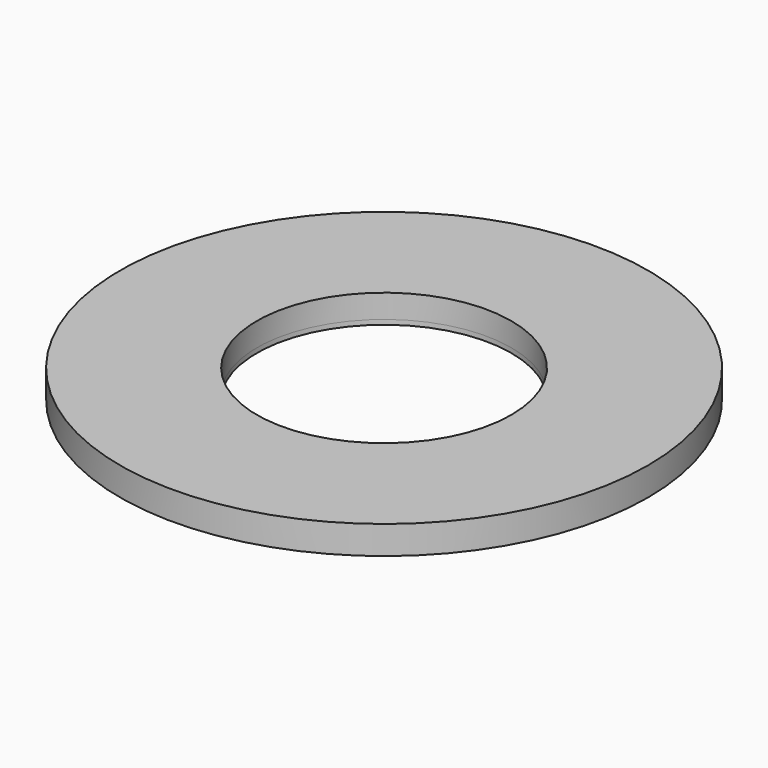
from build123d import *

# Parameters (mm, degrees)
F1_DEPTH      = 12.7
F0_W          = 50.8
F0_H          = 76.2
F0_W_2        = 25.4
F0_H_2        = 50.8
F2_R          = 177.8
F2_R_2        = 85.725
F3_DEPTH      = 15.875
F3_DEPTH_BACK = 3.175


# Not quite as in the source:
# - a feature names something its author has since deleted; it is built from what else it names


with BuildPart() as f1:
    # F0 (on Top) → F1 (new body)
    with BuildSketch(Plane.XY):
        Polygon((-76.6013473564, 51.7745457072), (-37.6862896459, 84.4281562793), (-86.666705504, 142.800742845), (-125.5817632145, 110.1471322729), align=None)
        Polygon((-107.6895961438, 108.5817704883), (-88.2320672886, 124.9085757744), (-55.5784567165, 85.9935180639), (-75.0359855718, 69.6667127779), align=None, mode=Mode.SUBTRACT)
    extrude(amount=F1_DEPTH)


with BuildPart() as f1b:
    # F0 (on Top) → F1, piece 2 (new body)
    with BuildSketch(Plane.XY):
        with Locations((0, 127)):
            Rectangle(F0_W, F0_H)
        with Locations((0, 127)):
            Rectangle(F0_W_2, F0_H_2, mode=Mode.SUBTRACT)
    extrude(amount=F1_DEPTH)


with BuildPart() as f1c:
    # F0 (on Top) → F1, piece 3 (new body)
    with BuildSketch(Plane.XY):
        Polygon((-91.9600729555, -9.5767939319), (-83.13874553, 40.4514399211), (-158.1810963096, 53.6834310593), (-167.0024237351, 3.6551972063), align=None)
        Polygon((-152.2900334154, 13.9569238132), (-147.8793697027, 38.9710407397), (-97.8511358497, 30.1497133142), (-102.2617995624, 5.1355963877), align=None, mode=Mode.SUBTRACT)
    extrude(amount=F1_DEPTH)


with BuildPart() as f1d:
    # F0 (on Top) → F1, piece 4 (new body)
    with BuildSketch(Plane.XY):
        Polygon((37.6862896459, 84.4281562793), (76.6013473564, 51.7745457072), (125.5817632145, 110.1471322729), (86.666705504, 142.800742845), align=None)
        Polygon((88.2320672886, 124.9085757744), (107.6895961438, 108.5817704883), (75.0359855718, 69.6667127779), (55.5784567165, 85.9935180639), align=None, mode=Mode.SUBTRACT)
    extrude(amount=F1_DEPTH)


with BuildPart() as f1e:
    # F0 (on Top) → F1, piece 5 (new body)
    with BuildSketch(Plane.XY):
        Polygon((83.13874553, 40.4514399211), (91.9600729555, -9.5767939319), (167.0024237351, 3.6551972063), (158.1810963096, 53.6834310593), align=None)
        Polygon((147.8793697027, 38.9710407397), (152.2900334154, 13.9569238132), (102.2617995624, 5.1355963877), (97.8511358497, 30.1497133142), align=None, mode=Mode.SUBTRACT)
    extrude(amount=F1_DEPTH)


with BuildPart() as f1f:
    # F0 (on Top) → F1, piece 6 (new body)
    with BuildSketch(Plane.XY):
        Polygon((89.6896583964, -22.4529547439), (64.2896583964, -66.4470452561), (130.2807941648, -104.5470452561), (155.6807941648, -60.5529547439), align=None)
        Polygon((138.3322715367, -65.2014773719), (125.6322715367, -87.1985226281), (81.6381810245, -61.7985226281), (94.3381810245, -39.8014773719), align=None, mode=Mode.SUBTRACT)
    extrude(amount=F1_DEPTH)


with BuildPart() as f1g:
    # F0 (on Top) → F1, piece 7 (new body)
    with BuildSketch(Plane.XY):
        Polygon((54.2737833096, -74.8513623474), (6.5373981737, -92.2259856283), (32.5993330951, -163.8305633322), (80.335718231, -146.4559400513), align=None)
        Polygon((64.0579661268, -138.8654995875), (40.1897735589, -147.552811228), (22.8151502779, -99.8164260921), (46.6833428459, -91.1291144516), align=None, mode=Mode.SUBTRACT)
    extrude(amount=F1_DEPTH)


with BuildPart() as f1h:
    # F0 (on Top) → F1, piece 8 (new body)
    with BuildSketch(Plane.XY):
        Polygon((-6.5373981737, -92.2259856283), (-54.2737833096, -74.8513623474), (-80.335718231, -146.4559400513), (-32.5993330951, -163.8305633322), align=None)
        Polygon((-40.1897735589, -147.552811228), (-64.0579661268, -138.8654995875), (-46.6833428459, -91.1291144516), (-22.8151502779, -99.8164260921), align=None, mode=Mode.SUBTRACT)
    extrude(amount=F1_DEPTH)


with BuildPart() as f1i:
    # F0 (on Top) → F1, piece 9 (new body)
    with BuildSketch(Plane.XY):
        Polygon((-64.2896583964, -66.4470452561), (-89.6896583964, -22.4529547439), (-155.6807941648, -60.5529547439), (-130.2807941648, -104.5470452561), align=None)
        Polygon((-125.6322715367, -87.1985226281), (-138.3322715367, -65.2014773719), (-94.3381810245, -39.8014773719), (-81.6381810245, -61.7985226281), align=None, mode=Mode.SUBTRACT)
    extrude(amount=F1_DEPTH)


with BuildPart() as f3:
    # F2 (on Top) → F3 (new body, two sides)
    with BuildSketch(Plane.XY) as f3_sk:
        Circle(F2_R)
        Circle(F2_R_2, mode=Mode.SUBTRACT)
    extrude(amount=F3_DEPTH)
    extrude(f3_sk.sketch, amount=-F3_DEPTH_BACK)


solid = Compound([f1.part, f1b.part, f1c.part, f1d.part, f1e.part, f1f.part, f1g.part, f1h.part, f1i.part, f3.part])
